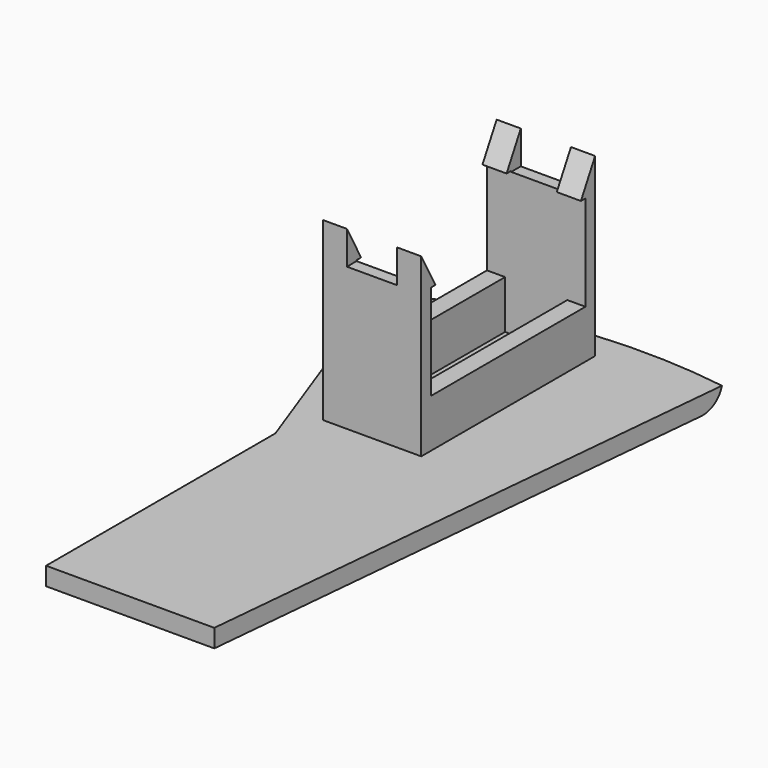
from build123d import *

# Parameters (mm, degrees)
F1_DEPTH    = 3.81
F3_T2_ANGLE = 45.4323000541
F2_W        = 20.7137
F2_H        = 2.54
F4_DEPTH    = 30.226
F8_DEPTH    = 20.7137
F9_W        = 10.5537
F9_H        = 7.0042966513
F10_DEPTH   = 51.8170001
F6_W        = 3.81
F6_H        = 40.64
F11_DEPTH   = 10.16


# Not quite as in the source:
# - a fillet or chamfer that OpenCascade refuses, or shapes differently, is made with other operations: its cross-section is extruded or revolved along the edge and cut away or added


with BuildPart() as f1:
    # F0 (on Top) → F1 (new body)
    with BuildSketch(Plane.XY):
        with BuildLine():
            ThreePointArc((32.3535154368, 26.1046796118), (-0.7575616132, 26.3503201986), (-32.5620487044, 17.1373747646))
            Line((-32.5620487044, 17.1373747646), (32.3535154368, 26.1046796118))
        make_face()
        Polygon((32.3535154368, 26.1046796118), (-32.5620487044, 17.1373747646), (-14.3325939581, -32.94764052), (-14.3325939581, -93.2497044648), (21.0546860419, -93.2497044648), align=None)
    extrude(amount=F1_DEPTH)

    # F3: fillet of radius 5.08 on 1 edges, made by hand

    # F3_s1 → F3_t2 (revolve, cut)
    with BuildSketch(Plane(origin=(35.6245782938, -9.4464852648, 0), x_dir=(0, 0, 1), z_dir=(0.966594728, -0.2563096405, 0))):
        with BuildLine():
            ThreePointArc((3.81, -34.1830353327), (1.0639073716, -32.3751984564), (0, -29.2643464831))
            Line((0, -29.2643464831), (0, -34.1830353327))
            Line((0, -34.1830353327), (3.81, -34.1830353327))
        make_face()
    revolve(axis=Axis((14.9550445097, -87.395415893, 0), (0, 0, 1)), revolution_arc=F3_T2_ANGLE, mode=Mode.SUBTRACT)

    # F2 (on face) → F4 (join)
    with BuildSketch(Plane.XY.offset(3.81)):
        with Locations((-0.8633345632, 20.0644456113)):
            Rectangle(F2_W, F2_H)
        with Locations((-0.8633345632, -23.1155543887)):
            Rectangle(F2_W, F2_H)
    extrude(amount=F4_DEPTH)

    # F7 (on face) → F8 (join)
    with BuildSketch(Plane.YZ.offset(9.4935154368)):
        Polygon((-24.3855543887, 40.8603511751), (-24.3855543887, 34.036), (-21.8455543887, 34.036), (-20.6579078442, 34.036), align=None)
        Polygon((17.6067990667, 34.036), (21.3344456113, 34.036), (21.3344456113, 40.8603511751), align=None)
    extrude(amount=-F8_DEPTH)

    # F9 (on face) → F10 (cut, through all)
    with BuildSketch(Plane.XZ.offset(24.3855543887)):
        with Locations((-0.8633345632, 37.3582028494)):
            Rectangle(F9_W, F9_H)
    extrude(amount=-F10_DEPTH, mode=Mode.SUBTRACT)

    # F6 (on face) → F11 (join)
    with BuildSketch(Plane.XY.offset(3.81)):
        with Locations((7.5885154368, -1.5255543887)):
            Rectangle(F6_W, F6_H)
        with Locations((-9.3151845632, -1.5255543887)):
            Rectangle(F6_W, F6_H)
    extrude(amount=F11_DEPTH)


solid = f1.part
